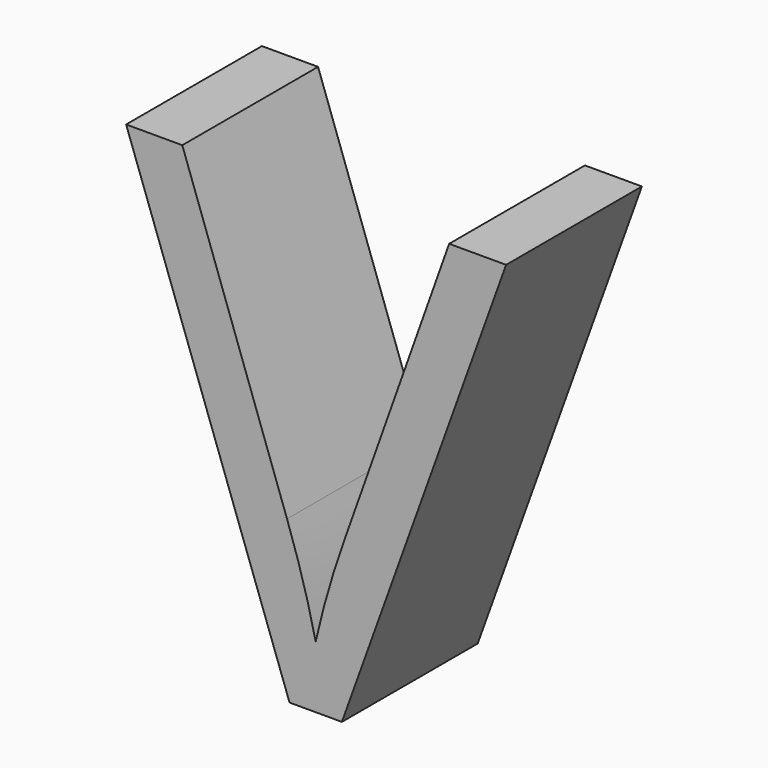
from build123d import *

# Parameters (mm, degrees)
F0_TEXT_SIZE = 94.0378755331
F1_DEPTH     = 25


# Not quite as in the source:
# - Text() gives the source's letters only with a copy of the font that has no kerning and outlines rounded to 1/6400 em; it was checked with that copy


with BuildPart() as f1:
    # F0 (on Front) → F1 (new body)
    with BuildSketch(Plane.XZ):
        with Locations((-49.410186708, -31.8402163684)):
            Text('V', F0_TEXT_SIZE, font='Open Sans', text_align=(TextAlign.LEFT, TextAlign.BOTTOM))
    extrude(amount=F1_DEPTH)


solid = f1.part
